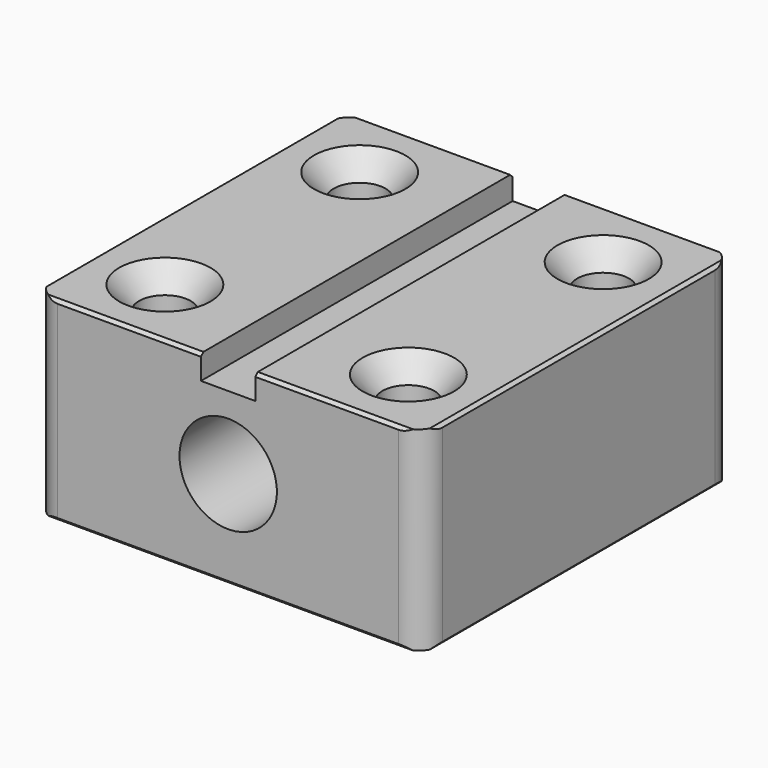
from build123d import *

# Parameters (mm, degrees)
F1_DEPTH       = 50.8
F3_D           = 13.49248
F3_CSINK_D     = 23.8252
F3_CSINK_ANGLE = 82
F4_SIZE        = 0.8128
F5_T1_DEPTH    = 80.9244
F7_D           = 25.4


# Not quite as in the source:
# - a fillet or chamfer that OpenCascade refuses, or shapes differently, is made with other operations: its cross-section is extruded or revolved along the edge and cut away or added


with BuildPart() as f1:
    # F0 (on Front) → F1 (new body, symmetric)
    with BuildSketch(Plane.XZ):
        Polygon((-7.0944838226, 25.4), (-50.8, 25.4), (-50.8, -25.4), (50.8, -25.4), (50.8, 25.4), (7.0944838226, 25.4), (7.0944838226, 19.05), (0, 19.05), (-7.0944838226, 19.05), align=None)
    extrude(amount=F1_DEPTH, both=True)

    # F3 (through all)
    with Locations(Plane.XY.offset(25.4)):
        with Locations((-31.75, 31.75), (31.75, 31.75), (31.75, -31.75), (-31.75, -31.75)):
            CounterSinkHole(F3_D / 2, F3_CSINK_D / 2, counter_sink_angle=F3_CSINK_ANGLE)

    # F4
    f4_edges = [f1.edges().sort_by_distance(p)[0] for p in [
        (-50.8, 0, 25.4),
        (50.8, 0, 25.4),
        (0, -50.8, -25.4),
        (-50.8, 0, -25.4),
        (0, 50.8, -25.4),
        (50.8, 0, -25.4),
        (-28.947242, -50.8, 25.4),
        (28.947242, -50.8, 25.4),
        (28.947242, 50.8, 25.4),
        (-28.947242, 50.8, 25.4),
    ]]
    chamfer(f4_edges, length=F4_SIZE)

    # F5: fillet of radius 6.35 on 4 edges, made by hand

    # F5_s2 → F5_t1 (cut)
    with BuildSketch(Plane.XY.offset(-40.4622)):
        with BuildLine():
            ThreePointArc((-44.45, -50.8), (-48.9401280605, -48.9401280605), (-50.8, -44.45))
            Line((-50.8, -44.45), (-50.8, -50.8))
            Line((-50.8, -50.8), (-44.45, -50.8))
        make_face()
        with BuildLine():
            ThreePointArc((44.45, -50.8), (48.9401280605, -48.9401280605), (50.8, -44.45))
            Line((50.8, -44.45), (50.8, -50.8))
            Line((50.8, -50.8), (44.45, -50.8))
        make_face()
        with BuildLine():
            ThreePointArc((44.45, 50.8), (48.9401280605, 48.9401280605), (50.8, 44.45))
            Line((50.8, 44.45), (50.8, 50.8))
            Line((50.8, 50.8), (44.45, 50.8))
        make_face()
        with BuildLine():
            ThreePointArc((-44.45, 50.8), (-48.9401280605, 48.9401280605), (-50.8, 44.45))
            Line((-50.8, 44.45), (-50.8, 50.8))
            Line((-50.8, 50.8), (-44.45, 50.8))
        make_face()
    extrude(amount=F5_T1_DEPTH, mode=Mode.SUBTRACT)

    # F7 (through all)
    with Locations(Plane.XZ.offset(50.8)):
        with Locations((0, 0)):
            Hole(F7_D / 2)


solid = f1.part
